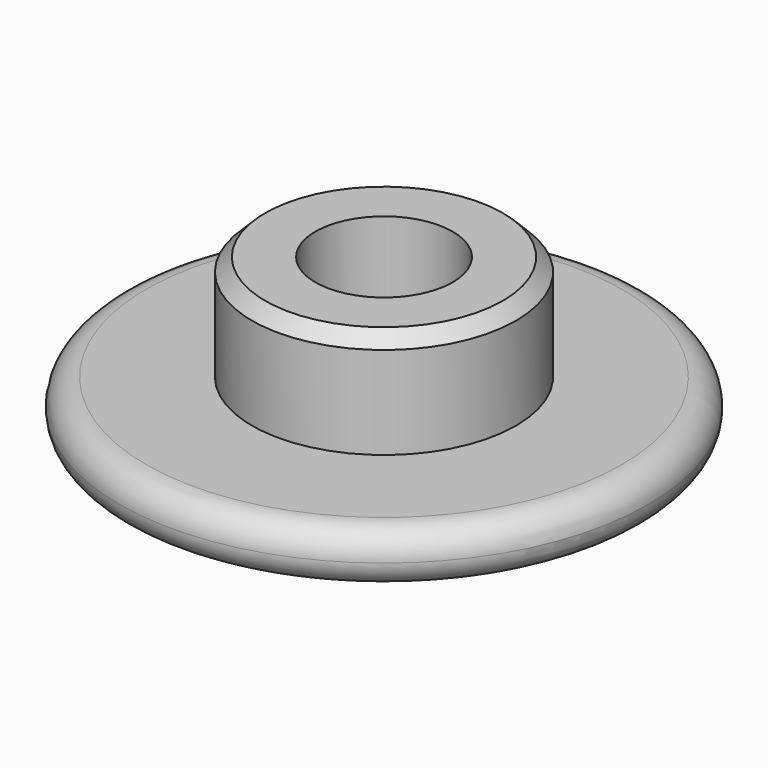
from build123d import *

# Parameters (mm, degrees)
F0_R     = 10
F1_DEPTH = 2
F2_R     = 5
F3_DEPTH = 4
F4_SIZE  = 0.5
F5_R     = 0.99999
F6_R     = 2.6
F7_DEPTH = 3.4


# Not quite as in the source:
# - a fillet or chamfer is up to 0.001 mm smaller than in the source, because OpenCascade refuses the exact size


with BuildPart() as f1:
    # F0 (on Top) → F1 (new body)
    with BuildSketch(Plane.XY):
        Circle(F0_R)
    extrude(amount=F1_DEPTH)

    # F2 (on face) → F3 (join)
    with BuildSketch(Plane.XY.offset(2)):
        Circle(F2_R)
    extrude(amount=F3_DEPTH)

    # F4
    f4_edges = [f1.edges().sort_by_distance(p)[0] for p in [
        (-5, 0, 6),
    ]]
    chamfer(f4_edges, length=F4_SIZE)

    # F5 (radius 1 in the source; OpenCascade refuses exactly that, so slightly less here)
    f5_edges = [f1.edges().sort_by_distance(p)[0] for p in [
        (-10, 0, 0),
        (-10, 0, 2),
    ]]
    fillet(f5_edges, radius=F5_R)

    # F6 (on face) → F7 (cut)
    with BuildSketch(Plane.XY.offset(6)):
        Circle(F6_R)
    extrude(amount=-F7_DEPTH, mode=Mode.SUBTRACT)


solid = f1.part
